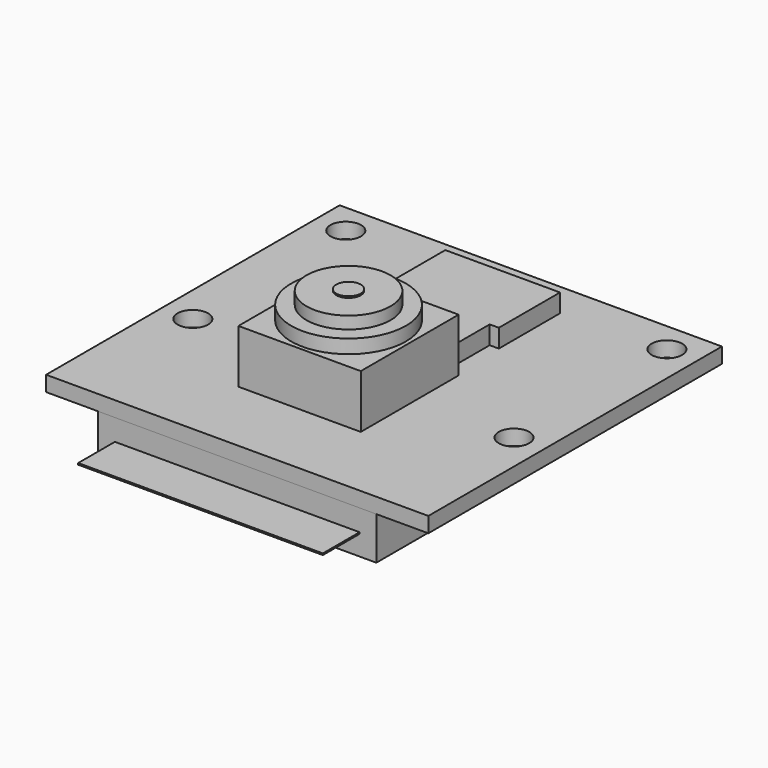
from build123d import *

# Parameters (mm, degrees)
F0_W      = 25
F0_H      = 24
F0_R      = 1
F1_DEPTH  = 1
F2_R      = 3.75
F2_R_2    = 2.75
F3_DEPTH  = 3.5
F4_DEPTH  = 4.4
F5_DEPTH  = 5.2
F6_R      = 0.8
F7_DEPTH  = 0.1
F8_W      = 18.2
F8_H      = 5.6
F9_DEPTH  = 2.8
F11_DEPTH = 1.2
F13_W     = 16
F13_H     = 3
F14_DEPTH = 0.1


with BuildPart() as f1:
    # F0 (on Top) → F1 (new body)
    with BuildSketch(Plane.XY):
        Rectangle(F0_W, F0_H)
        with Locations((-10.5, -2.5)):
            Circle(F0_R, mode=Mode.SUBTRACT)
        with Locations((10.5, -2.5)):
            Circle(F0_R, mode=Mode.SUBTRACT)
        with Locations((-10.5, 10)):
            Circle(F0_R, mode=Mode.SUBTRACT)
        with Locations((10.5, 10)):
            Circle(F0_R, mode=Mode.SUBTRACT)
    extrude(amount=F1_DEPTH)


with BuildPart() as f3:
    # F2 (on face) → F3 (new body)
    with BuildSketch(Plane.XY.offset(1)):
        Polygon((4, -6.9), (4, 1.1), (3.4, 1.1), (-3.4, 1.1), (-4, 1.1), (-4, -6.9), align=None)
        with Locations((0, -2.9)):
            Circle(F2_R, mode=Mode.SUBTRACT)
        with Locations((0, -2.9)):
            Circle(F2_R)
        with Locations((0, -2.9)):
            Circle(F2_R_2, mode=Mode.SUBTRACT)
        with Locations((0, -2.9)):
            Circle(F2_R_2)
    extrude(amount=F3_DEPTH)

    # F2 (on face) → F4 (join)
    with BuildSketch(Plane.XY.offset(1)):
        with Locations((0, -2.9)):
            Circle(F2_R)
        with Locations((0, -2.9)):
            Circle(F2_R_2, mode=Mode.SUBTRACT)
        with Locations((0, -2.9)):
            Circle(F2_R_2)
    extrude(amount=F4_DEPTH)

    # F2 (on face) → F5 (join)
    with BuildSketch(Plane.XY.offset(1)):
        with Locations((0, -2.9)):
            Circle(F2_R_2)
    extrude(amount=F5_DEPTH)


with BuildPart() as f7:
    # F6 (on face) → F7 (new body)
    with BuildSketch(Plane.XY.offset(6.2)):
        with Locations((0, -2.9)):
            Circle(F6_R)
    extrude(amount=F7_DEPTH)


with BuildPart() as f9:
    # F8 (on face) → F9 (new body)
    with BuildSketch(Plane(origin=(0, 0, 0), x_dir=(1, 0, 0), z_dir=(0, 0, -1))):
        with Locations((0, 9.2)):
            Rectangle(F8_W, F8_H)
    extrude(amount=F9_DEPTH)


with BuildPart() as f11:
    # F10 (on face) → F11 (new body)
    with BuildSketch(Plane.XY.offset(1)):
        Polygon((-3.15, 4.7), (-3.15, 1.1), (3.15, 1.1), (3.15, 4.7), (3.75, 4.7), (3.75, 9.7), (-3.75, 9.7), (-3.75, 4.7), align=None)
    extrude(amount=F11_DEPTH)


with BuildPart() as f14:
    # F13 (on offset) → F14 (new body)
    with BuildSketch(Plane(origin=(0, 0, -1.4), x_dir=(1, 0, 0), z_dir=(0, 0, -1))):
        with Locations((0, 13.5)):
            Rectangle(F13_W, F13_H)
    extrude(amount=F14_DEPTH)


solid = Compound([f1.part, f3.part, f7.part, f9.part, f11.part, f14.part])
